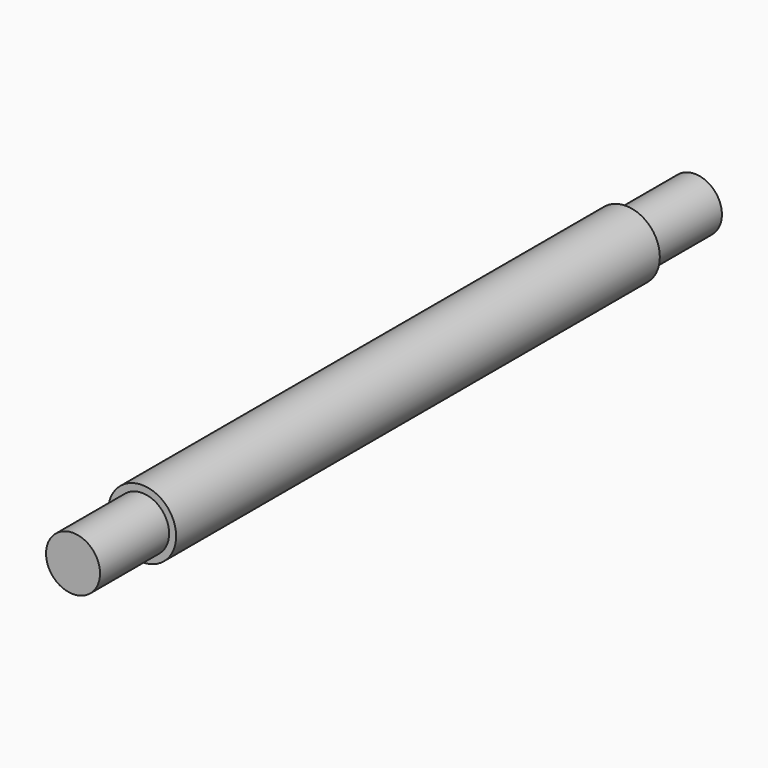
from build123d import *

# Parameters (mm, degrees)
F0_R     = 3.15
F1_DEPTH = 28
F2_R     = 2.5
F3_DEPTH = 8


# Not quite as in the source:
# - a pattern or mirror of a feature is missing from the dataset's text; its kind, count and spacing are read off the source's solid


with BuildPart() as f1:
    # F0 (on Front) → F1 (new body, symmetric)
    with BuildSketch(Plane.XZ):
        Circle(F0_R)
    extrude(amount=F1_DEPTH, both=True)

    # F2 (on face) → F3 (join)
    with BuildSketch(Plane.XZ.offset(28)):
        Circle(F2_R)
    f3 = extrude(amount=F3_DEPTH)

    # F3_copies: F3 across plane
    add(f3.mirror(Plane.ZX))


solid = f1.part
